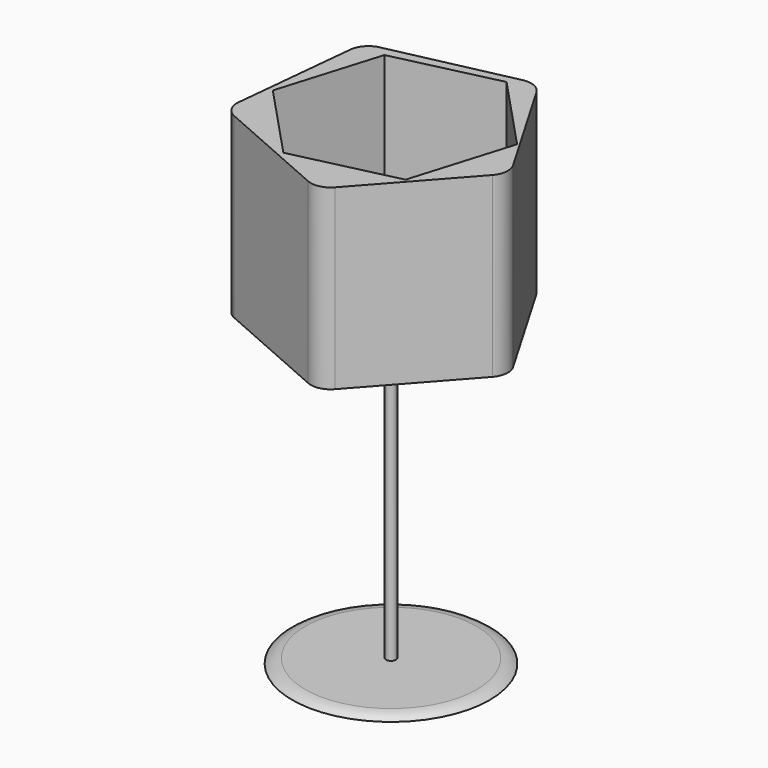
from build123d import *

# Parameters (mm, degrees)
F0_R     = 25.4
F1_DEPTH = 1.27
F3_R     = 1.27
F4_DEPTH = 76.2
F5_R     = 1.27
F6_DEPTH = 45.72
F8_DEPTH = 44.45
F9_R     = 5.08
F10_R    = 5.08
F11_R    = 5.08
F12_R    = 5.08
F13_R    = 5.08


# Not quite as in the source:
# - a fillet or chamfer that OpenCascade refuses, or shapes differently, is made with other operations: its cross-section is extruded or revolved along the edge and cut away or added


with BuildPart() as f1:
    # F0 (on Top) → F1 (new body)
    with BuildSketch(Plane.XY):
        Circle(F0_R)
    extrude(amount=F1_DEPTH)

    # F2: fillet of radius 5.08 on 1 edges, made by hand

    # F2_s1 → F2_t2 (revolve, cut)
    with BuildSketch(Plane.XZ):
        with BuildLine():
            ThreePointArc((25.4, 0), (23.8359470592, 0.9419048812), (22.0398958349, 1.27))
            Line((22.0398958349, 1.27), (25.4, 1.27))
            Line((25.4, 1.27), (25.4, 0))
        make_face()
    revolve(axis=Axis((0, 0, 1.27), (0, 0, 1)), mode=Mode.SUBTRACT)

    # F3 (on face) → F4 (join)
    with BuildSketch(Plane.XY.offset(1.27)):
        Circle(F3_R)
    extrude(amount=F4_DEPTH)


with BuildPart() as f6:
    # F5 (on face) → F6 (new body)
    with BuildSketch(Plane.XY.offset(77.47)):
        Polygon((7.1284634836, -32.8111068162), (33.4080333046, -3.3596179632), (13.5188365959, 30.7347487257), (-25.0529328, 22.3547373114), (-29.0024005842, -16.9187612577), align=None)
        Circle(F5_R, mode=Mode.SUBTRACT)
    extrude(amount=F6_DEPTH)

    # F7 (on face) → F8 (cut)
    with BuildSketch(Plane.XY.offset(123.19)):
        Polygon((18.5908850385, -18.5730540045), (26.4800313758, 7.4486517199), (7.8891463373, 27.2917057244), (-18.5908850385, 21.1130540045), (-26.4800313758, -4.9086517199), (-7.8891463373, -24.7517057244), align=None)
    extrude(amount=-F8_DEPTH, mode=Mode.SUBTRACT)

    # F9
    f9_edges = [f6.edges().sort_by_distance(p)[0] for p in [
        (33.408033, -3.359618, 100.33),
    ]]
    fillet(f9_edges, radius=F9_R)

    # F10
    f10_edges = [f6.edges().sort_by_distance(p)[0] for p in [
        (7.128463, -32.811107, 100.33),
    ]]
    fillet(f10_edges, radius=F10_R)

    # F11
    f11_edges = [f6.edges().sort_by_distance(p)[0] for p in [
        (-29.002401, -16.918761, 100.33),
    ]]
    fillet(f11_edges, radius=F11_R)

    # F12
    f12_edges = [f6.edges().sort_by_distance(p)[0] for p in [
        (-25.052933, 22.354737, 100.33),
    ]]
    fillet(f12_edges, radius=F12_R)

    # F13
    f13_edges = [f6.edges().sort_by_distance(p)[0] for p in [
        (13.518837, 30.734749, 100.33),
    ]]
    fillet(f13_edges, radius=F13_R)


solid = Compound([f1.part, f6.part])
